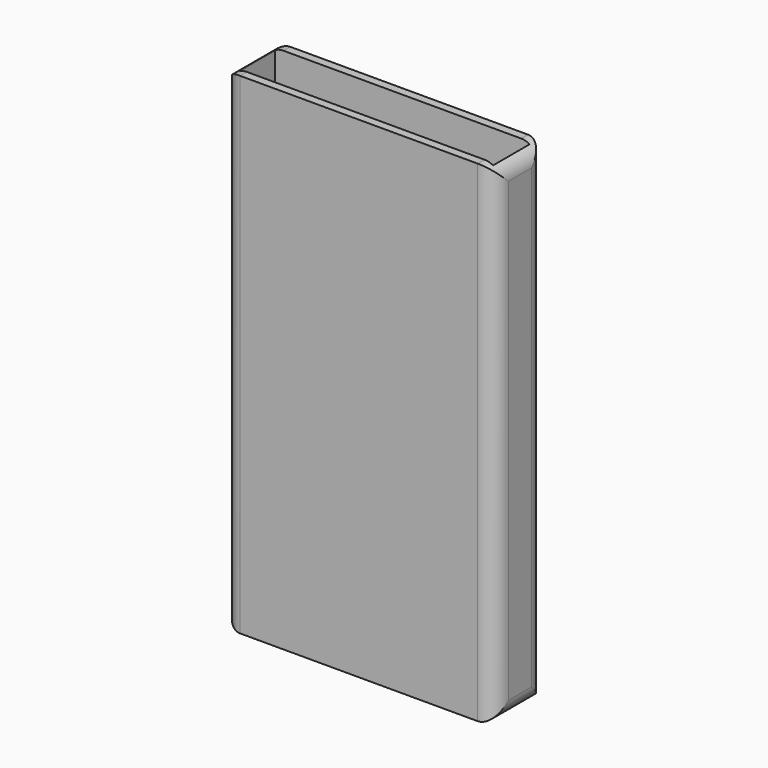
from build123d import *

# Parameters (mm, degrees)
F0_W        = 80
F0_H        = 144.526
F1_DEPTH    = 18.5
F2_T        = -2.5
F3_T1_DEPTH = 169.526
F3_T3_DEPTH = 43.5


# Not quite as in the source:
# - a fillet or chamfer that OpenCascade refuses, or shapes differently, is made with other operations: its cross-section is extruded or revolved along the edge and cut away or added


with BuildPart() as f1:
    # F0 (on Front) → F1 (new body)
    with BuildSketch(Plane.XZ):
        with Locations((4.5181000233, 3.1507380013)):
            Rectangle(F0_W, F0_H)
    extrude(amount=F1_DEPTH)

    # F2
    f2_openings = [f1.faces().sort_by_distance(p)[0] for p in [
        (4.5181, -9.25, 75.413738),
    ]]
    offset(amount=F2_T, openings=f2_openings)

    # F3: fillet of radius 5 on 8 edges, made by hand

    # F3_s2 → F3_t1 (cut)
    with BuildSketch(Plane.XY.offset(-81.6122619987)):
        with BuildLine():
            ThreePointArc((-35.4818999767, -13.5), (-34.0174338827, -17.0355339059), (-30.4818999767, -18.5))
            Line((-30.4818999767, -18.5), (-35.4818999767, -18.5))
            Line((-35.4818999767, -18.5), (-35.4818999767, -13.5))
        make_face()
        with BuildLine():
            ThreePointArc((-35.4818999767, -5), (-34.0174338827, -1.4644660941), (-30.4818999767, 0))
            Line((-30.4818999767, 0), (-35.4818999767, 0))
            Line((-35.4818999767, 0), (-35.4818999767, -5))
        make_face()
        with BuildLine():
            ThreePointArc((44.5181000233, -13.5), (43.0536339292, -17.0355339059), (39.5181000233, -18.5))
            Line((39.5181000233, -18.5), (44.5181000233, -18.5))
            Line((44.5181000233, -18.5), (44.5181000233, -13.5))
        make_face()
        with BuildLine():
            ThreePointArc((44.5181000233, -5), (43.0536339292, -1.4644660941), (39.5181000233, 0))
            Line((39.5181000233, 0), (44.5181000233, 0))
            Line((44.5181000233, 0), (44.5181000233, -5))
        make_face()
    extrude(amount=F3_T1_DEPTH, mode=Mode.SUBTRACT)

    # F3_s4 → F3_t3 (cut)
    with BuildSketch(Plane.XZ.offset(-12.5)):
        with BuildLine():
            ThreePointArc((44.5181000233, 70.4137380013), (43.0536339292, 73.9492719073), (39.5181000233, 75.4137380013))
            Line((39.5181000233, 75.4137380013), (44.5181000233, 75.4137380013))
            Line((44.5181000233, 75.4137380013), (44.5181000233, 70.4137380013))
        make_face()
        with BuildLine():
            ThreePointArc((-35.4818999767, 70.4137380013), (-34.0174338827, 73.9492719073), (-30.4818999767, 75.4137380013))
            Line((-30.4818999767, 75.4137380013), (-35.4818999767, 75.4137380013))
            Line((-35.4818999767, 75.4137380013), (-35.4818999767, 70.4137380013))
        make_face()
        with BuildLine():
            ThreePointArc((-35.4818999767, -64.1122619987), (-34.0174338827, -67.6477959046), (-30.4818999767, -69.1122619987))
            Line((-30.4818999767, -69.1122619987), (-35.4818999767, -69.1122619987))
            Line((-35.4818999767, -69.1122619987), (-35.4818999767, -64.1122619987))
        make_face()
        with BuildLine():
            ThreePointArc((39.5181000233, -69.1122619987), (43.0536339292, -67.6477959046), (44.5181000233, -64.1122619987))
            Line((44.5181000233, -64.1122619987), (44.5181000233, -69.1122619987))
            Line((44.5181000233, -69.1122619987), (39.5181000233, -69.1122619987))
        make_face()
    extrude(amount=F3_T3_DEPTH, mode=Mode.SUBTRACT)


solid = f1.part
